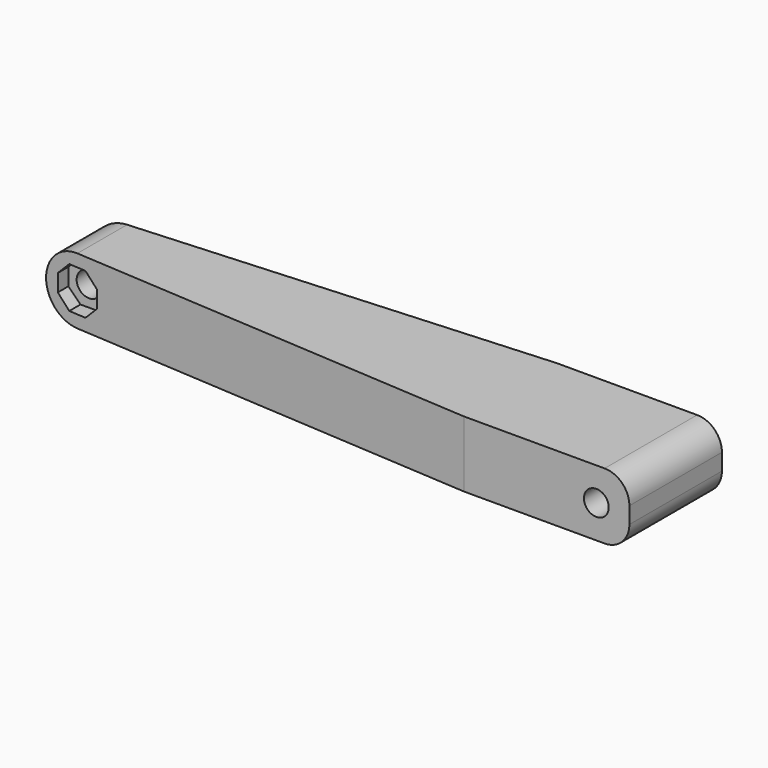
from build123d import *

# Parameters (mm, degrees)
F0_W      = 36.7
F0_H      = 7
F1_DEPTH  = 4
F3_R      = 0.75
F4_DEPTH  = 25
F5_R      = 1.99999
F6_R      = 0.75
F7_DEPTH  = 25
F8_R      = 1.5
F9_R      = 0.75
F10_DEPTH = 2.5
F11_DEPTH = 25


# Not quite as in the source:
# - a fillet or chamfer is up to 0.001 mm smaller than in the source, because OpenCascade refuses the exact size


with BuildPart() as f1:
    # F0 (on Top) → F1 (new body)
    with BuildSketch(Plane.XY):
        with Locations((-18.35, -3.5)):
            Rectangle(F0_W, F0_H)
    extrude(amount=F1_DEPTH)

    # F3 (on face) → F4 (cut)
    with BuildSketch(Plane(origin=(0, 0, 0), x_dir=(-1, 0, 0), z_dir=(0, 1, 0))):
        with Locations((2, 2)):
            Circle(F3_R)
    extrude(amount=-F4_DEPTH, mode=Mode.SUBTRACT)

    # F5 (radius 2 in the source; OpenCascade refuses exactly that, so slightly less here)
    f5_edges = [f1.edges().sort_by_distance(p)[0] for p in [
        (-36.7, -3.5, 0),
        (-36.7, -3.5, 4),
    ]]
    fillet(f5_edges, radius=F5_R)

    # F6 (on face) → F7 (cut)
    with BuildSketch(Plane(origin=(0, 0, 0), x_dir=(-1, 0, 0), z_dir=(0, 1, 0))):
        with Locations((34.7, 2)):
            Circle(F6_R)
    extrude(amount=-F7_DEPTH, mode=Mode.SUBTRACT)

    # F8
    f8_edges = [f1.edges().sort_by_distance(p)[0] for p in [
        (0, -3.5, 4),
        (0, -3.5, 0),
    ]]
    fillet(f8_edges, radius=F8_R)

    # F9 (on face) → F10 (cut)
    with BuildSketch(Plane.XZ.offset(7)):
        Polygon((-33.45, 1.482233047), (-33.45, 2.517766953), (-34.182233047, 3.25), (-35.217766953, 3.25), (-35.95, 2.517766953), (-35.95, 1.482233047), (-35.217766953, 0.75), (-34.182233047, 0.75), align=None)
        with Locations((-34.7, 2)):
            Circle(F9_R, mode=Mode.SUBTRACT)
    extrude(amount=-F10_DEPTH, mode=Mode.SUBTRACT)

    # F2 (on face) → F11 (cut)
    with BuildSketch(Plane.XY.offset(4)):
        Polygon((-36.7, 0), (-36.7, -1.75), (-10, 0), align=None)
        Polygon((-10, -7), (-36.7, -5.25), (-36.7, -7), align=None)
    extrude(amount=-F11_DEPTH, mode=Mode.SUBTRACT)


solid = f1.part
